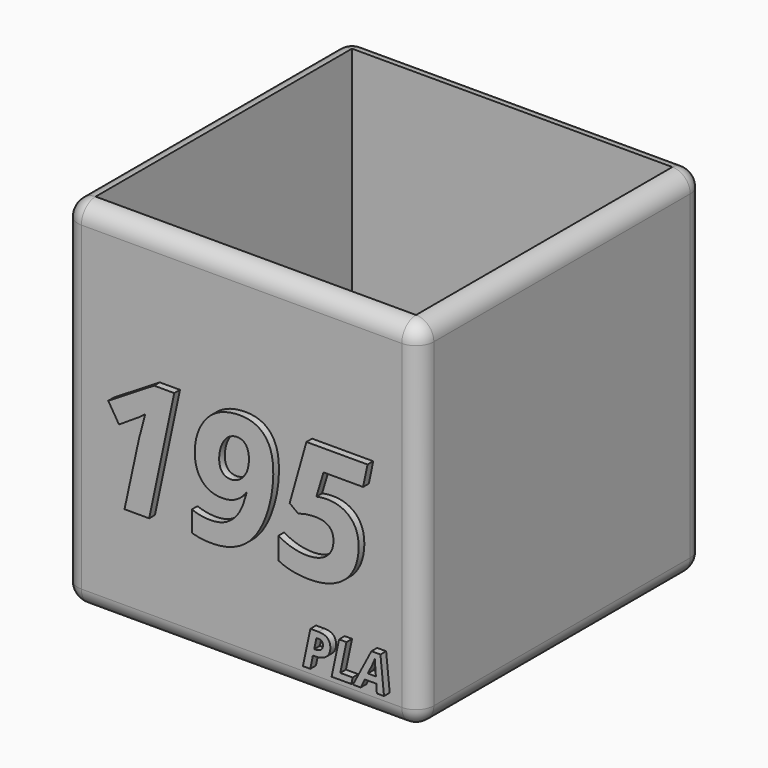
from build123d import *

# Parameters (mm, degrees)
F0_W         = 20
F0_H         = 20
F1_DEPTH     = 20
F2_R         = 1
F3_T         = 1
F4_R         = 0.99999
F7_TEXT_SIZE = 9.3175614195
F8_DEPTH     = 0.4
F9_TEXT_SIZE = 2.7777777778
F10_DEPTH    = 0.4


# Not quite as in the source:
# - a fillet or chamfer is up to 0.001 mm smaller than in the source, because OpenCascade refuses the exact size
# - a shell that OpenCascade refuses in one call is made with other operations: the cavity is built on its own and cut out
# - Text() gives the source's letters only with a copy of the font that has no kerning and outlines rounded to 1/6400 em; it was checked with that copy


with BuildPart() as f1:
    # F0 (on Top) → F1 (new body)
    with BuildSketch(Plane.XY):
        Rectangle(F0_W, F0_H)
    extrude(amount=F1_DEPTH)

    # F2
    f2_edges = [f1.edges().sort_by_distance(p)[0] for p in [
        (10, 10, 10),
        (-10, -10, 10),
        (10, -10, 10),
        (-10, 10, 10),
        (10, 0, 0),
        (0, -10, 0),
        (0, 10, 0),
        (-10, 0, 0),
    ]]
    fillet(f2_edges, radius=F2_R)

    # F3: shell of thickness 1, made by hand


with BuildPart() as f3_core1:
    # F3_t2: copy of F1
    add(f1.part)

    # the walls: a layer under each face that stays
    f3_faces = [f3_core1.faces().sort_by_distance(p)[0] for p in [
        (0, -10, 10.5),
        (-10, 0, 10.5),
        (10, 0, 10.5),
        (0, 10, 10.5),
        (0, 0, 0),
    ]]
    thicken(f3_faces, amount=-F3_T, mode=Mode.SUBTRACT)


with BuildPart() as f1_1:
    add(f1.part)

    # what is left inside the walls is the cavity
    f3_cavity = [f3_core1.part.solids().sort_by_distance(p)[0] for p in [
        (-8.99, 0, 13.666667),
    ]]
    add(f3_cavity, mode=Mode.SUBTRACT)

    # F4 (radius 1 in the source; OpenCascade refuses exactly that, so slightly less here)
    f4_edges = [f1_1.edges().sort_by_distance(p)[0] for p in [
        (9.707107, 9.707107, 20),
        (-9.707107, 9.707107, 20),
        (0, -10, 20),
        (0, 10, 20),
        (-9.707107, -9.707107, 20),
        (10, 0, 20),
        (-10, 0, 20),
        (9.707107, -9.707107, 20),
    ]]
    fillet(f4_edges, radius=F4_R)

    # F7 (on face) → F8 (join)
    with BuildSketch(Plane.XZ.offset(10)):
        with Locations((-8, 6)):
            Text('195', F7_TEXT_SIZE, font='Open Sans', font_style=FontStyle.BOLDITALIC, text_align=(TextAlign.LEFT, TextAlign.BOTTOM))
    extrude(amount=F8_DEPTH)

    # F9 (on face) → F10 (join)
    with BuildSketch(Plane.XZ.offset(10)):
        with Locations((3.6918402778, 1.5)):
            Text('PLA', F9_TEXT_SIZE, font='Open Sans', font_style=FontStyle.BOLDITALIC, text_align=(TextAlign.LEFT, TextAlign.BOTTOM))
    extrude(amount=F10_DEPTH)


solid = f1_1.part
